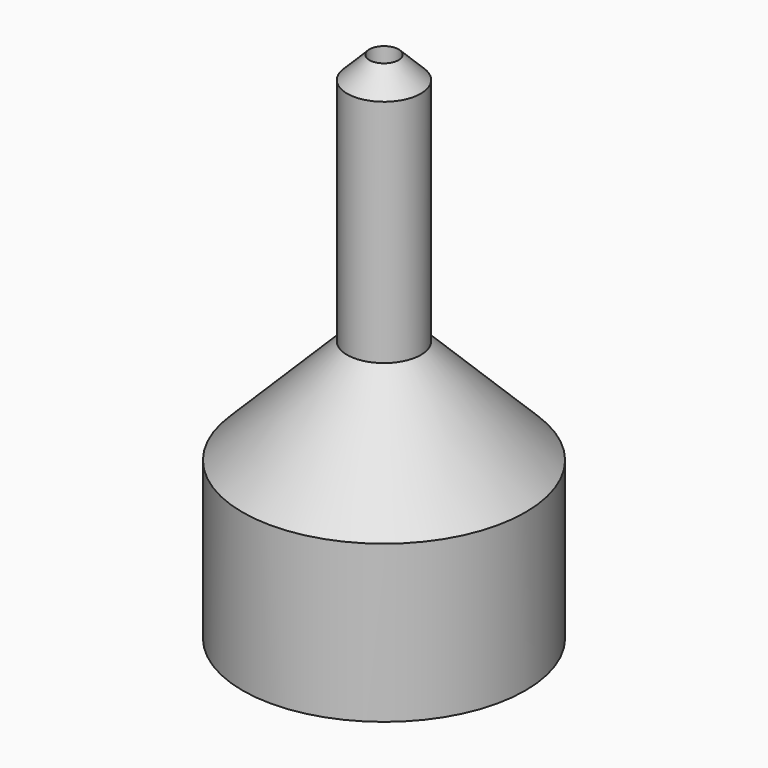
from build123d import *

# Parameters (mm, degrees)
F0_R     = 13.5257644579
F1_DEPTH = 25
F2_SIZE  = 10
F3_DEPTH = 25
F4_R     = 1.3988438113
F5_DEPTH = 100


# Not quite as in the source:
# - a fillet or chamfer that OpenCascade refuses, or shapes differently, is made with other operations: its cross-section is extruded or revolved along the edge and cut away or added


with BuildPart() as f1:
    # F0 (on Top) → F1 (new body)
    with BuildSketch(Plane.XY):
        Circle(F0_R)
    extrude(amount=F1_DEPTH)

    # F2
    f2_edges = [f1.edges().sort_by_distance(p)[0] for p in [
        (-13.525764, 0, 25),
    ]]
    chamfer(f2_edges, length=F2_SIZE)

    # F3 (add): a face of the model
    f3_faces = [f1.faces().sort_by_distance(p)[0] for p in [
        (0, 0, 25),
    ]]
    extrude(f3_faces, amount=F3_DEPTH)

    # F4 (on face) → F5 (cut)
    with BuildSketch(Plane.XY.offset(50)):
        Circle(F4_R)
    extrude(amount=-F5_DEPTH, mode=Mode.SUBTRACT)

    # F6: chamfer of 3 on 1 edges, made by hand

    # F6_s1 → F6_t2 (revolve, cut)
    with BuildSketch(Plane.XZ):
        Polygon((3.5257644579, 47), (0.5257644579, 50), (3.5257644579, 50), align=None)
    revolve(axis=Axis((0, 0, 50), (0, 0, 1)), mode=Mode.SUBTRACT)


solid = f1.part
